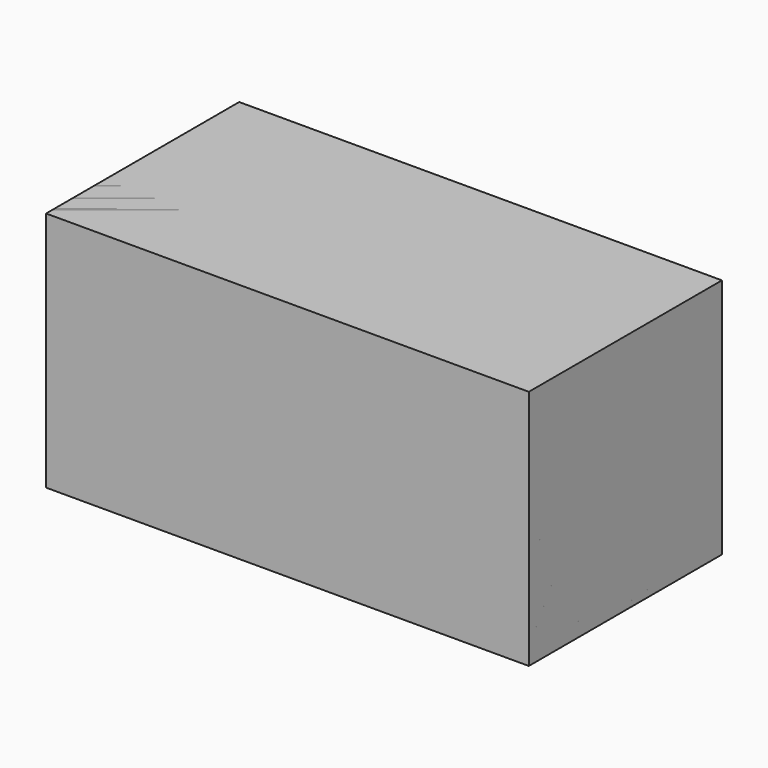
from build123d import *

# Parameters (mm, degrees)
F0_W            = 100
F0_H            = 50
F1_DEPTH        = 50
F3_DEPTH        = 96
F6_DEPTH        = 25
F8_DEPTH        = 46
F10_DEPTH       = 46
F13_DEPTH       = 25
F16_DEPTH       = 25
F17_TEXT_SIZE   = 8.3333333333
F17_TEXT_SIZE_2 = 11.1111111111
F18_DEPTH       = 1
F19_TEXT_SIZE   = 8.3333333333
F19_TEXT_SIZE_2 = 11.1111111111
F20_DEPTH       = 1
F21_TEXT_SIZE   = 8.3333333333
F21_TEXT_SIZE_2 = 11.1111111111
F22_DEPTH       = 1
F23_TEXT_SIZE   = 8.3333333333
F23_TEXT_SIZE_2 = 11.1111111111
F24_DEPTH       = 1
F25_TEXT_SIZE   = 8.3333333333
F25_TEXT_SIZE_2 = 11.1111111111
F26_DEPTH       = 1
F27_TEXT_SIZE   = 8.3333333333
F27_TEXT_SIZE_2 = 11.1111111111
F28_DEPTH       = 1
F29_W           = 100
F29_H           = 50
F30_DEPTH       = 50


# Not quite as in the source:
# - Text() gives the source's letters only with a copy of the font that has no kerning and outlines rounded to 1/6400 em; it was checked with that copy


with BuildPart() as f1:
    # F0 (on Top) → F1 (new body)
    with BuildSketch(Plane.XY):
        with Locations((50, 25)):
            Rectangle(F0_W, F0_H)
    extrude(amount=F1_DEPTH)

    # F2 (on face) → F3 (cut, through all)
    with BuildSketch(Plane(origin=(0, 0, 0), x_dir=(0, -1, 0), z_dir=(-1, 0, 0))):
        Polygon((0, 0), (0, 2), (-2, 0), align=None)
    extrude(amount=-F3_DEPTH, mode=Mode.SUBTRACT)

    # F5 (on 3pt) → F6 (cut)
    with BuildSketch(Plane(origin=(11.1111111111, 22.2222222222, 22.2222222222), x_dir=(-0.9428090416, 0.2357022604, 0.2357022604), z_dir=(0.3333333333, 0.6666666667, 0.6666666667))):
        Polygon((-90.0382634711, -1.4142135624), (-90.0382634711, 1.4142135624), (-94.2809041582, 0), align=None)
    extrude(amount=-F6_DEPTH, mode=Mode.SUBTRACT)

    # F7 (on face) → F8 (cut)
    with BuildSketch(Plane.XZ):
        Polygon((0, 2), (0, 0), (2, 0), align=None)
    extrude(amount=-F8_DEPTH, mode=Mode.SUBTRACT)

    # F9 (on face) → F10 (cut)
    with BuildSketch(Plane(origin=(0, 0, 0), x_dir=(1, 0, 0), z_dir=(0, 0, -1))):
        Polygon((0, -2), (2, 0), (0, 0), align=None)
    extrude(amount=-F10_DEPTH, mode=Mode.SUBTRACT)

    # F12 (on 3pt) → F13 (cut)
    with BuildSketch(Plane(origin=(11.1111111111, 11.1111111111, 5.5555555556), x_dir=(-0.7453559925, 0.596284794, 0.298142397), z_dir=(0.6666666667, 0.6666666667, 0.3333333333))):
        Polygon((14.90711985, 40.249223595), (14.90711985, 44.72135955), (12.223838277, 41.143650786), align=None)
    extrude(amount=-F13_DEPTH, mode=Mode.SUBTRACT)

    # F15 (on 3pt) → F16 (cut)
    with BuildSketch(Plane(origin=(11.1111111111, 5.5555555556, 11.1111111111), x_dir=(0.7453559925, -0.298142397, -0.596284794), z_dir=(-0.6666666667, -0.3333333333, -0.6666666667))):
        Polygon((-12.223838277, -41.143650786), (-14.90711985, -40.249223595), (-14.90711985, -44.72135955), align=None)
    extrude(amount=F16_DEPTH, mode=Mode.SUBTRACT)

    # F17 (on face) → F18 (cut)
    with BuildSketch(Plane.XZ):
        Polygon((47, 40), (22, 40), (22, 15), (24, 19), (24, 38), (43, 38), align=None)
        with Locations((19.6506702913, 7.8810919598)):
            Text('Y', F17_TEXT_SIZE, font='Open Sans', font_style=FontStyle.BOLD, text_align=(TextAlign.LEFT, TextAlign.BOTTOM))
        with Locations((48.4343486561, 35.9369265437)):
            Text('X', F17_TEXT_SIZE, font='Open Sans', font_style=FontStyle.BOLD, text_align=(TextAlign.LEFT, TextAlign.BOTTOM))
        with Locations((26.2137199618, 28.2547654659)):
            Text('F', F17_TEXT_SIZE_2, font='Open Sans', font_style=FontStyle.BOLD, text_align=(TextAlign.LEFT, TextAlign.BOTTOM))
        with Locations((3.2918651123, 42.3296103776)):
            Text('Z', F17_TEXT_SIZE, font='Open Sans', font_style=FontStyle.BOLD, text_align=(TextAlign.LEFT, TextAlign.BOTTOM))
        with Locations((91.6254743934, 3.8148966208)):
            Text('X', F17_TEXT_SIZE, font='Open Sans', font_style=FontStyle.BOLD, text_align=(TextAlign.LEFT, TextAlign.BOTTOM))
    extrude(amount=-F18_DEPTH, mode=Mode.SUBTRACT)

    # F19 (on face) → F20 (cut)
    with BuildSketch(Plane(origin=(0, 0, 0), x_dir=(1, 0, 0), z_dir=(0, 0, -1))):
        Polygon((47, -12.8631396219), (22, -12.8631396219), (22, -37.8631396219), (24, -33.8631396219), (24, -14.8631396219), (43, -14.8631396219), align=None)
        with Locations((20.2276314609, -45.1056122507)):
            Text('Y', F19_TEXT_SIZE, font='Open Sans', font_style=FontStyle.BOLD, text_align=(TextAlign.LEFT, TextAlign.BOTTOM))
        with Locations((48.5593259418, -16.5194937686)):
            Text('X', F19_TEXT_SIZE, font='Open Sans', font_style=FontStyle.BOLD, text_align=(TextAlign.LEFT, TextAlign.BOTTOM))
        with Locations((91.4665752451, -10.6068699347)):
            Text('X', F19_TEXT_SIZE, font='Open Sans', font_style=FontStyle.BOLD, text_align=(TextAlign.LEFT, TextAlign.BOTTOM))
        with Locations((27.1102438858, -25.1601735055)):
            Text('C', F19_TEXT_SIZE_2, font='Open Sans', font_style=FontStyle.BOLD, text_align=(TextAlign.LEFT, TextAlign.BOTTOM))
        with Locations((3.9556137328, -48.5298959017)):
            Text('Y', F19_TEXT_SIZE, font='Open Sans', font_style=FontStyle.BOLD, text_align=(TextAlign.LEFT, TextAlign.BOTTOM))
    extrude(amount=-F20_DEPTH, mode=Mode.SUBTRACT)

    # F21 (on face) → F22 (cut)
    with BuildSketch(Plane.XY.offset(50)):
        Polygon((47, 39.5129099488), (22, 39.5129099488), (22, 14.5129099488), (24, 18.5129099488), (24, 37.5129099488), (43, 37.5129099488), align=None)
        with Locations((19.9133659714, 6.8403842201)):
            Text('Y', F21_TEXT_SIZE, font='Open Sans', font_style=FontStyle.BOLD, text_align=(TextAlign.LEFT, TextAlign.BOTTOM))
        with Locations((49.0099221551, 35.7406499137)):
            Text('X', F21_TEXT_SIZE, font='Open Sans', font_style=FontStyle.BOLD, text_align=(TextAlign.LEFT, TextAlign.BOTTOM))
        with Locations((26.2350832766, 27.2622047067)):
            Text('E', F21_TEXT_SIZE_2, font='Open Sans', font_style=FontStyle.BOLD, text_align=(TextAlign.LEFT, TextAlign.BOTTOM))
    extrude(amount=-F22_DEPTH, mode=Mode.SUBTRACT)

    # F23 (on face) → F24 (cut)
    with BuildSketch(Plane(origin=(0, 50, 0), x_dir=(-1, 0, 0), z_dir=(0, 1, 0))):
        Polygon((-22, 9.3699758872), (-22, 34.3699758872), (-24, 30.3699758872), (-24, 11.3699758872), (-43, 11.3699758872), (-47, 9.3699758872), align=None)
        with Locations((-53.7769813091, 7.073774986)):
            Text('X', F23_TEXT_SIZE, font='Open Sans', font_style=FontStyle.BOLD, text_align=(TextAlign.LEFT, TextAlign.BOTTOM))
        with Locations((-25.7017990379, 35.4048880339)):
            Text('Y', F23_TEXT_SIZE, font='Open Sans', font_style=FontStyle.BOLD, text_align=(TextAlign.LEFT, TextAlign.BOTTOM))
        with Locations((-33.6396085629, 12.7336694002)):
            Text('D', F23_TEXT_SIZE_2, font='Open Sans', font_style=FontStyle.BOLD, text_align=(TextAlign.LEFT, TextAlign.BOTTOM))
    extrude(amount=-F24_DEPTH, mode=Mode.SUBTRACT)

    # F25 (on face) → F26 (cut)
    with BuildSketch(Plane(origin=(0, 0, 0), x_dir=(0, -1, 0), z_dir=(-1, 0, 0))):
        Polygon((-10.2241784334, 8.6948111653), (-10.2241784334, 33.6948111653), (-12.2241784334, 29.6948111653), (-12.2241784334, 10.6948111653), (-31.2241784334, 10.6948111653), (-35.2241784334, 8.6948111653), align=None)
        with Locations((-41.5607703278, 7.8786956357)):
            Text('X', F25_TEXT_SIZE, font='Open Sans', font_style=FontStyle.BOLD, text_align=(TextAlign.LEFT, TextAlign.BOTTOM))
        with Locations((-14.2701062538, 34.0699102009)):
            Text('Y', F25_TEXT_SIZE, font='Open Sans', font_style=FontStyle.BOLD, text_align=(TextAlign.LEFT, TextAlign.BOTTOM))
        with Locations((-22.315390408, 12.4237680882)):
            Text('A', F25_TEXT_SIZE_2, font='Open Sans', font_style=FontStyle.BOLD, text_align=(TextAlign.LEFT, TextAlign.BOTTOM))
        with Locations((-8.8645494353, 42)):
            Text('Z', F25_TEXT_SIZE, font='Open Sans', font_style=FontStyle.BOLD, text_align=(TextAlign.LEFT, TextAlign.BOTTOM))
        with Locations((-49.1289417397, 2.9824665338)):
            Text('Y', F25_TEXT_SIZE, font='Open Sans', font_style=FontStyle.BOLD, text_align=(TextAlign.LEFT, TextAlign.BOTTOM))
    extrude(amount=-F26_DEPTH, mode=Mode.SUBTRACT)

    # F27 (on face) → F28 (cut)
    with BuildSketch(Plane.YZ.offset(100)):
        Polygon((41.2107557058, 7.9915839015), (41.2107557058, 32.9915839015), (39.2107557058, 28.9915839015), (39.2107557058, 9.9915839015), (20.2107557058, 9.9915839015), (16.2107557058, 7.9915839015), align=None)
        with Locations((8.8477634465, 5.7702837723)):
            Text('X', F27_TEXT_SIZE, font='Open Sans', font_style=FontStyle.BOLD, text_align=(TextAlign.LEFT, TextAlign.BOTTOM))
        with Locations((37.0705873541, 33.6558851625)):
            Text('Y', F27_TEXT_SIZE, font='Open Sans', font_style=FontStyle.BOLD, text_align=(TextAlign.LEFT, TextAlign.BOTTOM))
        with Locations((29.3877553195, 11.7536638007)):
            Text('B', F27_TEXT_SIZE_2, font='Open Sans', font_style=FontStyle.BOLD, text_align=(TextAlign.LEFT, TextAlign.BOTTOM))
    extrude(amount=-F28_DEPTH, mode=Mode.SUBTRACT)


with BuildPart() as f30:
    # F29 (on Top) → F30 (new body)
    with BuildSketch(Plane.XY):
        with Locations((50, 25)):
            Rectangle(F29_W, F29_H)
    extrude(amount=F30_DEPTH)


solid = Compound([f1.part, f30.part])
